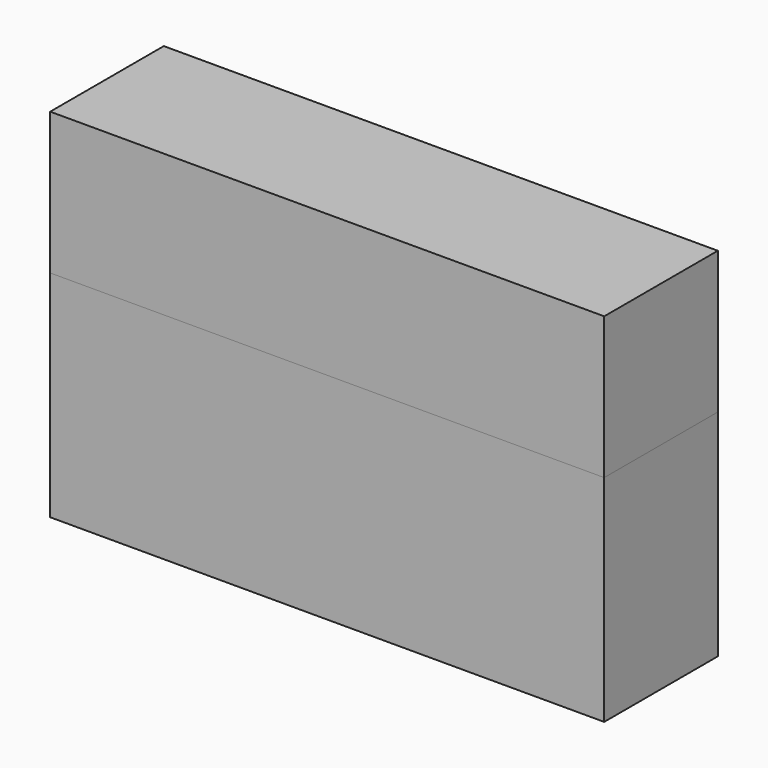
from build123d import *

# Parameters (mm, degrees)
F0_W     = 99.1016365588
F0_H     = 38.474753499
F1_DEPTH = 25.4
F2_DEPTH = 25.4


# Not quite as in the source:
# - a feature of the source that left no trace in its solid (it failed there, or was rolled back) is left out


with BuildPart() as f1:
    # F0 (on Front) → F1 (new body)
    with BuildSketch(Plane.XZ):
        with Locations((3.2062288374, -5.9752464294)):
            Rectangle(F0_W, F0_H)
    extrude(amount=F1_DEPTH)


with BuildPart() as f2:
    # F2 (new): a face of the model
    f2_faces = [f1.part.faces().sort_by_distance(p)[0] for p in [
        (3.2062288374, -12.7, 13.2621303201),
    ]]
    extrude(f2_faces, amount=F2_DEPTH)


solid = Compound([f1.part, f2.part])
